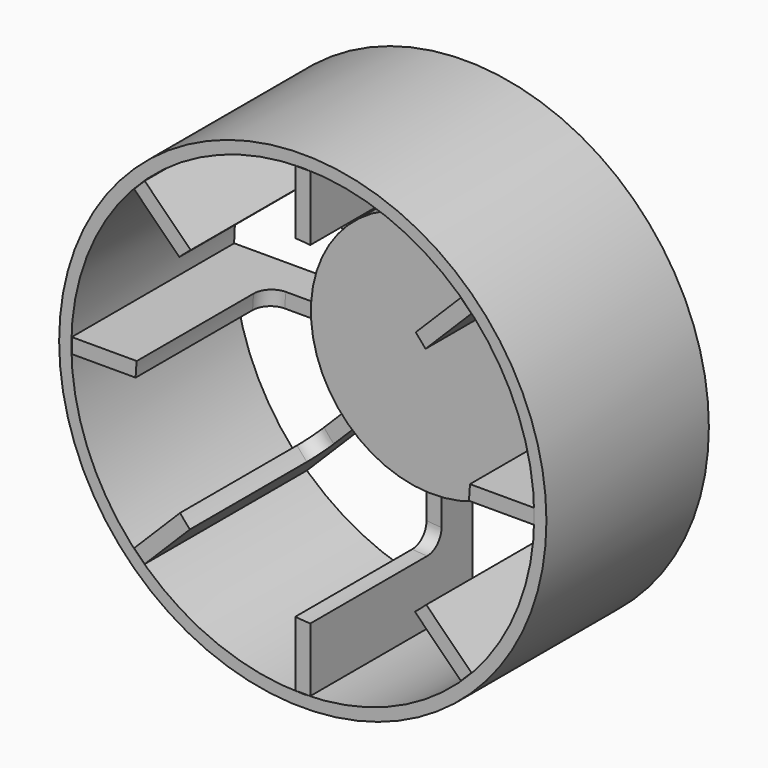
from build123d import *

# Parameters (mm, degrees)
F0_R      = 30
F1_DEPTH  = 25
F2_R      = 28.5
F3_DEPTH  = 43.4
F4_R      = 15
F5_DEPTH  = 5
F6_W      = 1.8436461687
F6_H      = 13.4322764352
F7_DEPTH  = 25
F8_R      = 24.1088040978
F9_DEPTH  = 20.2
F11_R     = 2.1969343418
F12_COUNT = 8


# Not quite as in the source:
# - a feature of the source that left no trace in its solid (it failed there, or was rolled back) is left out


with BuildPart() as f1:
    # F0 (on Front) → F1 (new body)
    with BuildSketch(Plane.XZ):
        Circle(F0_R)
    extrude(amount=F1_DEPTH)

    # F2 (on Front) → F3 (cut)
    with BuildSketch(Plane.XZ):
        Circle(F2_R)
    extrude(amount=F3_DEPTH, mode=Mode.SUBTRACT)


with BuildPart() as f5:
    # F4 (on Front) → F5 (new body)
    with BuildSketch(Plane.XZ):
        Circle(F4_R)
    extrude(amount=F5_DEPTH)


with BuildPart() as f7:
    # F6 (on Front) → F7 (new body)
    with BuildSketch(Plane.XZ):
        with Locations((1.164e-07, 21.7286809348)):
            Rectangle(F6_W, F6_H)
    extrude(amount=F7_DEPTH)

    # F8 (on face) → F9 (cut)
    with BuildSketch(Plane.XZ.offset(25)):
        with Locations((-1.7935009673, -3.5128288437)):
            Circle(F8_R)
    extrude(amount=-F9_DEPTH, mode=Mode.SUBTRACT)

    # F11
    f11_edges = [f7.edges().sort_by_distance(p)[0] for p in [
        (0.00132, -4.8, 20.529073),
    ]]
    fillet(f11_edges, radius=F11_R)


with BuildPart() as f12_1:
    # F12: instance of F7
    add(f7.part.rotate(Axis((0, 0, 0), (0, 1, 0)), 1 * 360 / F12_COUNT))


with BuildPart() as f12_2:
    # F12: instance of F7
    add(f7.part.rotate(Axis((0, 0, 0), (0, 1, 0)), 2 * 360 / F12_COUNT))


with BuildPart() as f12_3:
    # F12: instance of F7
    add(f7.part.rotate(Axis((0, 0, 0), (0, 1, 0)), 3 * 360 / F12_COUNT))


with BuildPart() as f12_4:
    # F12: instance of F7
    add(f7.part.rotate(Axis((0, 0, 0), (0, 1, 0)), 4 * 360 / F12_COUNT))


with BuildPart() as f12_5:
    # F12: instance of F7
    add(f7.part.rotate(Axis((0, 0, 0), (0, 1, 0)), 5 * 360 / F12_COUNT))


with BuildPart() as f12_6:
    # F12: instance of F7
    add(f7.part.rotate(Axis((0, 0, 0), (0, 1, 0)), 6 * 360 / F12_COUNT))


with BuildPart() as f12_7:
    # F12: instance of F7
    add(f7.part.rotate(Axis((0, 0, 0), (0, 1, 0)), 7 * 360 / F12_COUNT))


solid = Compound([f1.part, f5.part, f7.part, f12_1.part, f12_2.part, f12_3.part, f12_4.part, f12_5.part, f12_6.part, f12_7.part])
